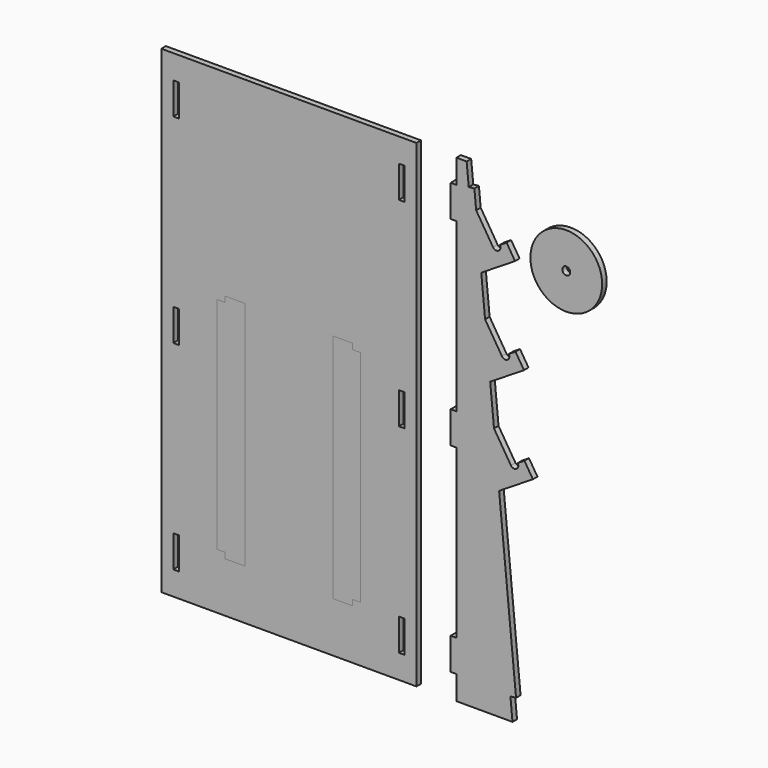
from build123d import *

# Parameters (mm, degrees)
F1_W     = 812.8
F1_H     = 1524
F1_W_2   = 18.034
F1_H_2   = 101.6
F2_DEPTH = 18.034
F1_R     = 114.3
F1_R_2   = 12.7
F1_W_3   = 63.5
F1_H_3   = 18.034
F3_DEPTH = 18.034


# Not quite as in the source:
# - a variable given as a bare number and used for a length is read in inches; the dataset says mm whatever the document's units were


with BuildPart() as f2:
    # F1 (on Front) → F2 (new body)
    with BuildSketch(Plane.XZ):
        Rectangle(F1_W, F1_H)
        with Locations((-359.283, -635)):
            Rectangle(F1_W_2, F1_H_2, mode=Mode.SUBTRACT)
        Polygon((-203.2, -584.2), (-228.6, -584.2), (-228.6, 116.332), (-203.2, 116.332), (-203.2, 134.366), (-139.7, 134.366), (-139.7, 116.332), (-139.7, -584.2), (-139.7, -602.234), (-203.2, -602.234), align=None, mode=Mode.SUBTRACT)
        Polygon((139.7, -602.234), (139.7, -584.2), (139.7, 116.332), (139.7, 134.366), (203.2, 134.366), (203.2, 116.332), (228.6, 116.332), (228.6, -584.2), (203.2, -584.2), (203.2, -602.234), align=None, mode=Mode.SUBTRACT)
        with Locations((359.283, -635)):
            Rectangle(F1_W_2, F1_H_2, mode=Mode.SUBTRACT)
        with Locations((-359.283, 0)):
            Rectangle(F1_W_2, F1_H_2, mode=Mode.SUBTRACT)
        with Locations((-359.283, 635)):
            Rectangle(F1_W_2, F1_H_2, mode=Mode.SUBTRACT)
        with Locations((359.283, 0)):
            Rectangle(F1_W_2, F1_H_2, mode=Mode.SUBTRACT)
        with Locations((359.283, 635)):
            Rectangle(F1_W_2, F1_H_2, mode=Mode.SUBTRACT)
    extrude(amount=F2_DEPTH)


with BuildPart() as f2b:
    # F1 (on Front) → F2, piece 2 (new body)
    with BuildSketch(Plane.XZ):
        with Locations((524.383, -635)):
            Rectangle(F1_W_2, F1_H_2)
        with Locations((524.383, 0)):
            Rectangle(F1_W_2, F1_H_2)
        with Locations((524.383, 635)):
            Rectangle(F1_W_2, F1_H_2)
        Polygon((650.269536136, 548.8751497174), (596.3708333333, 635), (607.2071109947, 521.9257983161), align=None)
        with BuildLine():
            Line((650.269536136, 548.8751497174), (607.2071109947, 521.9257983161))
            Line((607.2071109947, 521.9257983161), (612.6252498254, 465.3886974742))
            Line((612.6252498254, 465.3886974742), (720.2813126786, 532.7620759775))
            Line((720.2813126786, 532.7620759775), (693.3319612773, 575.8245011188))
            Line((693.3319612773, 575.8245011188), (671.8007487066, 562.3498254181))
            ThreePointArc((671.8007487066, 562.3498254181), (667.7724802716, 544.8468812825), (650.269536136, 548.8751497174))
        make_face()
        Polygon((678.6947859614, 252.2638471916), (624.7960831587, 338.3886974742), (635.6323608201, 225.3144957903), align=None)
        with BuildLine():
            Line((678.6947859614, 252.2638471916), (635.6323608201, 225.3144957903))
            Line((635.6323608201, 225.3144957903), (641.0504996508, 168.7773949484))
            Line((641.0504996508, 168.7773949484), (748.706562504, 236.1507734517))
            Line((748.706562504, 236.1507734517), (721.7572111026, 279.213198593))
            Line((721.7572111026, 279.213198593), (700.225998532, 265.7385228923))
            ThreePointArc((700.225998532, 265.7385228923), (696.197730097, 248.2355787566), (678.6947859614, 252.2638471916))
        make_face()
        Polygon((707.1200357868, -44.3474553342), (653.2213329841, 41.7773949484), (664.0576106455, -71.2968067355), align=None)
        with BuildLine():
            Line((664.0576106455, -71.2968067355), (669.4757494762, -127.8339075774))
            Line((669.4757494762, -127.8339075774), (777.1318123294, -60.4605290741))
            Line((777.1318123294, -60.4605290741), (750.182460928, -17.3981039329))
            Line((750.182460928, -17.3981039329), (728.6512483574, -30.8727796335))
            ThreePointArc((728.6512483574, -30.8727796335), (724.6229799224, -48.3757237692), (707.1200357868, -44.3474553342))
            Line((707.1200357868, -44.3474553342), (664.0576106455, -71.2968067355))
        make_face()
        Polygon((566.0833768912, 762), (533.4, 762), (533.4, 685.8), (533.4, 584.2), (533.4, 50.8), (533.4, -50.8), (533.4, -584.2), (533.4, -685.8), (533.4, -762), (712.1333768912, -762), (705.4699471859, -692.4685595967), (723.42170089, -690.7481832), (669.4757494762, -127.8339075774), (664.0576106455, -71.2968067355), (653.2213329841, 41.7773949484), (641.0504996508, 168.7773949484), (635.6323608201, 225.3144957903), (624.7960831587, 338.3886974742), (612.6252498254, 465.3886974742), (607.2071109947, 521.9257983161), (596.3708333333, 635), (590.6985603006, 694.1889359933), (572.7468065965, 692.4685595967), align=None)
    extrude(amount=F2_DEPTH)


with BuildPart() as f2c:
    # F1 (on Front) → F2, piece 3 (new body)
    with BuildSketch(Plane.XZ):
        with Locations((883.3532333374, 558.3602190018)):
            Circle(F1_R)
        with Locations((883.3532333374, 558.3602190018)):
            Circle(F1_R_2, mode=Mode.SUBTRACT)
    extrude(amount=F2_DEPTH)


with BuildPart() as f3:
    # F1 (on Front) → F3 (new body)
    with BuildSketch(Plane.XZ):
        Polygon((-228.6, 116.332), (-228.6, -584.2), (-203.2, -584.2), (-139.7, -584.2), (-139.7, 116.332), (-203.2, 116.332), align=None)
        with Locations((-171.45, 125.349)):
            Rectangle(F1_W_3, F1_H_3)
        with Locations((-171.45, -593.217)):
            Rectangle(F1_W_3, F1_H_3)
    extrude(amount=F3_DEPTH)


with BuildPart() as f3b:
    # F1 (on Front) → F3, piece 2 (new body)
    with BuildSketch(Plane.XZ):
        with Locations((171.45, 125.349)):
            Rectangle(F1_W_3, F1_H_3)
        Polygon((139.7, 116.332), (139.7, -584.2), (203.2, -584.2), (228.6, -584.2), (228.6, 116.332), (203.2, 116.332), align=None)
        with Locations((171.45, -593.217)):
            Rectangle(F1_W_3, F1_H_3)
    extrude(amount=F3_DEPTH)


solid = Compound([f2.part, f2b.part, f2c.part, f3.part, f3b.part])
